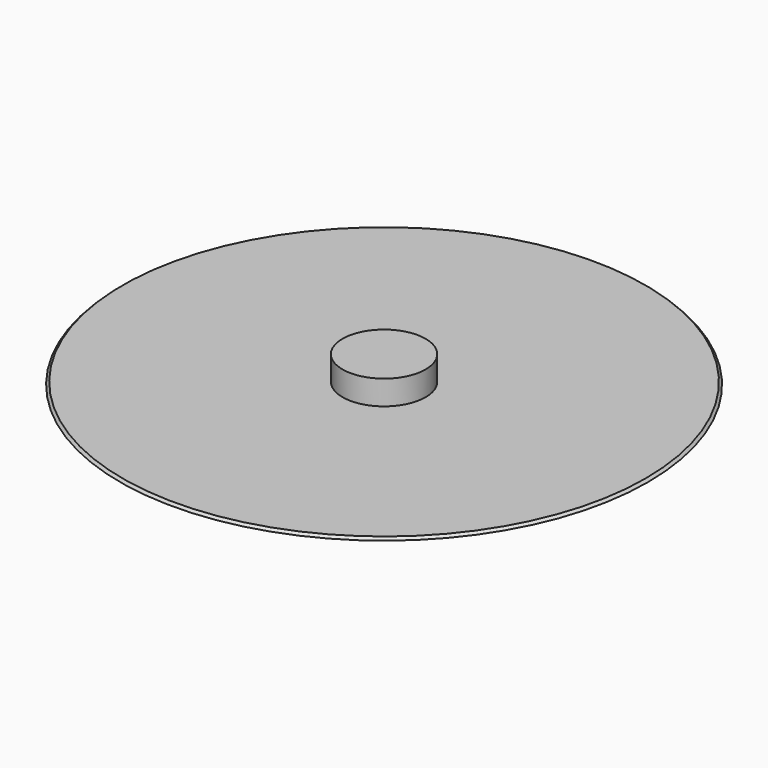
from build123d import *

# Parameters (mm, degrees)
F0_R     = 1371.6
F1_DEPTH = 12.7
F2_R     = 215.9
F3_DEPTH = 127
F4_SIZE  = 12.69999


# Not quite as in the source:
# - a fillet or chamfer is up to 0.001 mm smaller than in the source, because OpenCascade refuses the exact size


with BuildPart() as f1:
    # F0 (on Top) → F1 (new body)
    with BuildSketch(Plane.XY):
        Circle(F0_R)
    extrude(amount=F1_DEPTH)

    # F2 (on face) → F3 (join)
    with BuildSketch(Plane.XY.offset(12.7)):
        Circle(F2_R)
    extrude(amount=F3_DEPTH)

    # F4 (size 12.7 in the source; OpenCascade refuses exactly that, so slightly less here)
    f4_edges = [f1.edges().sort_by_distance(p)[0] for p in [
        (-1371.6, 0, 12.7),
    ]]
    chamfer(f4_edges, length=F4_SIZE)


solid = f1.part
